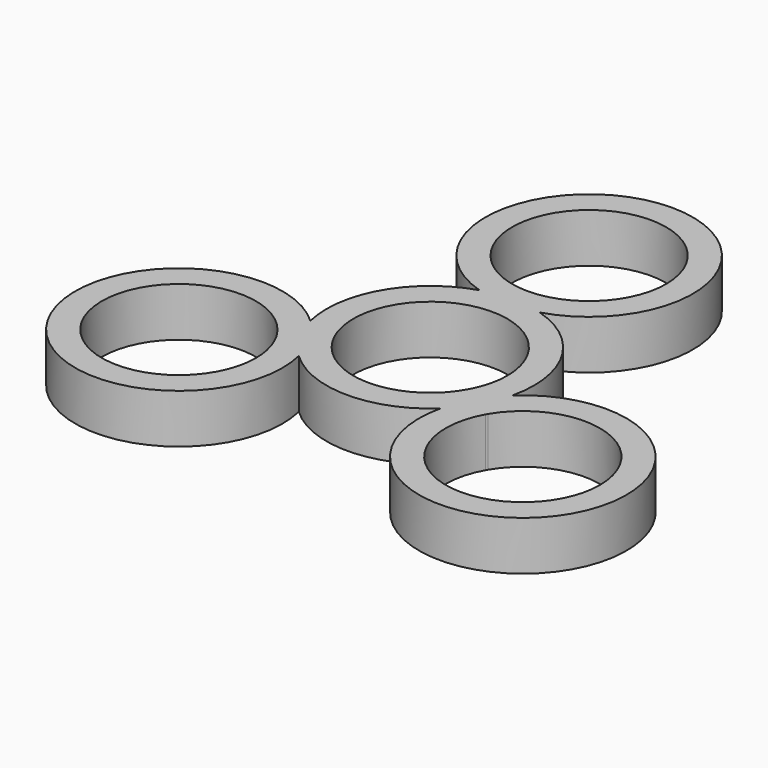
from build123d import *

# Parameters (mm, degrees)
F0_R     = 10.9982
F1_DEPTH = 7.0104
F4_DEPTH = 25.146


# Not quite as in the source:
# - a feature of the source that left no trace in its solid (it failed there, or was rolled back) is left out


with BuildPart() as f1:
    # F0 (on Top) → F1 (new body)
    with BuildSketch(Plane.XY):
        with BuildLine():
            ThreePointArc((17.2763619736, 1.5771367083), (15.0239819099, 8.6741), (10.0040214414, 14.1732))
            ThreePointArc((10.0040214414, 14.1732), (0, 45.6946), (-10.0040214414, 14.1732))
            ThreePointArc((-10.0040214414, 14.1732), (-15.0239819099, 8.6741), (-17.2763619736, 1.5771367083))
            ThreePointArc((-17.2763619736, 1.5771367083), (-39.5726844158, -22.8473), (-7.2723405322, -15.7503367083))
            ThreePointArc((-7.2723405322, -15.7503367083), (0, -17.3482), (7.2723405322, -15.7503367083))
            ThreePointArc((7.2723405322, -15.7503367083), (39.5726844158, -22.8473), (17.2763619736, 1.5771367083))
        make_face()
        with BuildLine():
            ThreePointArc((-13.5488898986, -14.1732), (-35.1543992189, -17.0912600791), (-15.0971116601, -8.5461841053))
            ThreePointArc((-15.0971116601, -8.5461841053), (-15.0225853511, -8.6732936964), (-14.9497683707, -8.8013901688))
            ThreePointArc((-14.9497683707, -8.8013901688), (-13.904869688, -11.3974658018), (-13.5488898986, -14.1732))
        make_face(mode=Mode.SUBTRACT)
        with BuildLine():
            ThreePointArc((15.0971116601, -8.5461841053), (27.466762585, -3.567503287), (35.5485151131, -14.1732))
            ThreePointArc((35.5485151131, -14.1732), (21.7729683076, -24.8170328179), (14.9497683707, -8.8013901688))
            ThreePointArc((14.9497683707, -8.8013901688), (15.0225853511, -8.6732936964), (15.0971116601, -8.5461841053))
        make_face(mode=Mode.SUBTRACT)
        Circle(F0_R, mode=Mode.SUBTRACT)
        with BuildLine():
            ThreePointArc((-0.1473432894, 17.3475742741), (-7.7257727387, 36.1763625148), (10.9998126072, 28.3464))
            ThreePointArc((10.9998126072, 28.3464), (7.8299625148, 20.6206272613), (0.1473432894, 17.3475742741))
            ThreePointArc((0.1473432894, 17.3475742741), (0, 17.3465873928), (-0.1473432894, 17.3475742741))
        make_face(mode=Mode.SUBTRACT)
    extrude(amount=F1_DEPTH)

    # F3 (on face) → F4 (cut)
    with BuildSketch(Plane(origin=(0, 0, 0), x_dir=(1, 0, 0), z_dir=(0, 0, -1))):
        with BuildLine():
            ThreePointArc((-10.0040214414, -14.1732), (0, -45.6946), (10.0040214414, -14.1732))
            ThreePointArc((10.0040214414, -14.1732), (15.0239819099, -8.6741), (17.2763619736, -1.5771367083))
            ThreePointArc((17.2763619736, -1.5771367083), (39.5726844158, 22.8473), (7.2723405322, 15.7503367083))
            ThreePointArc((7.2723405322, 15.7503367083), (0, 17.3482), (-7.2723405322, 15.7503367083))
            ThreePointArc((-7.2723405322, 15.7503367083), (-39.5726844158, 22.8473), (-17.2763619736, -1.5771367083))
            ThreePointArc((-17.2763619736, -1.5771367083), (-15.0239819099, -8.6741), (-10.0040214414, -14.1732))
        make_face()
        with BuildLine():
            ThreePointArc((10.1294026029, 10.8017600414), (37.3729807628, 21.5773005039), (14.4192999029, 3.3714399586))
            ThreePointArc((14.4192999029, 3.3714399586), (12.824278257, -7.4041005038), (4.2898973, -14.1732))
            ThreePointArc((4.2898973, -14.1732), (0, -43.1546010077), (-4.2898973, -14.1732))
            ThreePointArc((-4.2898973, -14.1732), (-12.824278257, -7.4041005038), (-14.4192999029, 3.3714399586))
            ThreePointArc((-14.4192999029, 3.3714399586), (-37.3729807628, 21.5773005038), (-10.1294026029, 10.8017600414))
            ThreePointArc((-10.1294026029, 10.8017600414), (0, 14.8082010077), (10.1294026029, 10.8017600414))
        make_face(mode=Mode.SUBTRACT)
    extrude(amount=-F4_DEPTH, mode=Mode.SUBTRACT)


solid = f1.part
